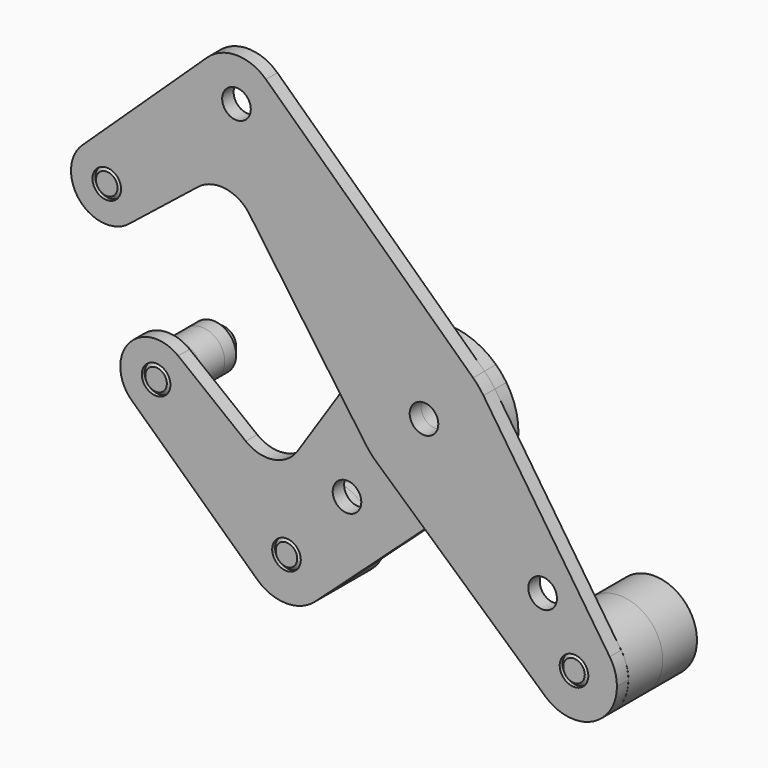
from build123d import *

# Parameters (mm, degrees)
F0_R      = 3.175
F0_R_2    = 3.96875
F2_DEPTH  = 3.175
F3_DEPTH  = 3.175
F4_R      = 9.525
F6_DEPTH  = 12.7
F4_R_2    = 5.08
F5_R      = 9.525
F5_R_2    = 5.08
F7_OFFSET = 0.0254
F8_SIZE   = 0.762
F8_2_SIZE = 0.762
F8_3_SIZE = 0.762
F8_4_SIZE = 0.762


with BuildPart() as f2:
    # F0 (on Front) → F2 (new body)
    with BuildSketch(Plane.XZ):
        with BuildLine():
            ThreePointArc((26.9262440233, -45.4676864135), (37.1682864336, -47.0737686401), (42.8102251661, -38.3762138003))
            ThreePointArc((42.8102251661, -38.3762138003), (42.3999454948, -35.6108027404), (41.2044512386, -33.0836262089))
            ThreePointArc((41.2044512386, -33.0836262089), (27.0442454474, -31.1806737127), (26.9262440233, -45.4676864135))
        make_face()
        with Locations((33.2852251661, -38.3762138003)):
            Circle(F0_R, mode=Mode.SUBTRACT)
        with BuildLine():
            ThreePointArc((-32.0815314576, 47.9702672503), (-32.8608164346, 51.7436071154), (-35.0711574392, 54.8995176744))
            ThreePointArc((-35.0711574392, 54.8995176744), (-41.6065314576, 57.4952672503), (-48.1419054761, 54.8995176744))
            ThreePointArc((-48.1419054761, 54.8995176744), (-45.3798713227, 39.2245522274), (-32.0815314576, 47.9702672503))
        make_face()
        with Locations((-41.6065314576, 47.9702672503)):
            Circle(F0_R, mode=Mode.SUBTRACT)
        with BuildLine():
            ThreePointArc((-62.4511918078, 23.0063483758), (-67.2442419203, 30.2944442282), (-75.8348368232, 28.7807237291))
            ThreePointArc((-75.8348368232, 28.7807237291), (-76.3849752141, 17.8055319436), (-65.4422370763, 16.798571653))
            ThreePointArc((-65.4422370763, 16.798571653), (-63.237943921, 19.5609585706), (-62.4511918078, 23.0063483758))
        make_face()
        with Locations((-70.3886918078, 23.0063483758)):
            Circle(F0_R, mode=Mode.SUBTRACT)
        with BuildLine():
            ThreePointArc((-12.9726166036, -9.1502373442), (-15.8730587934, -0.2482529814), (-13.2524193062, 8.7400805221))
            Line((-13.2524193062, 8.7400805221), (-19.2147683858, -0.3005169703))
            Line((-19.2147683858, -0.3005169703), (-12.9726166036, -9.1502373442))
        make_face()
        with BuildLine():
            Line((-10.5983019047, -11.8191210221), (0.0653932355, -21.3813431455))
            Line((0.0653932355, -21.3813431455), (10.6703987497, -11.7540722953))
            ThreePointArc((10.6703987497, -11.7540722953), (0.0485522706, -15.8749257534), (-10.5983019047, -11.8191210221))
        make_face()
        with BuildLine():
            ThreePointArc((26.9262440233, -45.4676864135), (27.0442454474, -31.1806737127), (41.2044512386, -33.0836262089))
            Line((41.2044512386, -33.0836262089), (13.1987101208, 8.820979319))
            ThreePointArc((13.1987101208, 8.820979319), (15.1912005478, 4.609018433), (15.875, 0))
            ThreePointArc((15.875, 0), (14.5156502636, -6.4274040191), (10.6703987497, -11.7540722953))
            Line((10.6703987497, -11.7540722953), (0.0653932355, -21.3813431455))
            Line((0.0653932355, -21.3813431455), (26.9262440233, -45.4676864135))
        make_face()
        with Locations((26.3222689506, -25.5025770961)):
            Circle(F0_R, mode=Mode.SUBTRACT)
        with BuildLine():
            ThreePointArc((-13.2524193062, 8.7400805221), (-1.834314477, 15.7686687897), (10.8922900307, 11.5487507067))
            Line((10.8922900307, 11.5487507067), (-35.0711574392, 54.8995176744))
            ThreePointArc((-35.0711574392, 54.8995176744), (-32.8608164346, 51.7436071154), (-32.0815314576, 47.9702672503))
            ThreePointArc((-32.0815314576, 47.9702672503), (-45.3798713227, 39.2245522274), (-48.1419054761, 54.8995176744))
            Line((-48.1419054761, 54.8995176744), (-75.8348368232, 28.7807237291))
            ThreePointArc((-75.8348368232, 28.7807237291), (-67.2442419203, 30.2944442282), (-62.4511918078, 23.0063483758))
            ThreePointArc((-62.4511918078, 23.0063483758), (-63.237943921, 19.5609585706), (-65.4422370763, 16.798571653))
            Line((-65.4422370763, 16.798571653), (-50.1509863937, 28.9828821829))
            ThreePointArc((-50.1509863937, 28.9828821829), (-44.0823996147, 30.6328866939), (-38.7182233604, 27.3502241323))
            Line((-38.7182233604, 27.3502241323), (-19.2147683858, -0.3005169703))
            Line((-19.2147683858, -0.3005169703), (-13.2524193062, 8.7400805221))
        make_face()
        with BuildLine():
            ThreePointArc((15.875, 0), (15.1912005478, 4.609018433), (13.1987101208, 8.820979319))
            ThreePointArc((13.1987101208, 8.820979319), (12.1224690662, 10.2499448164), (10.8922900307, 11.5487507067))
            ThreePointArc((10.8922900307, 11.5487507067), (-1.834314477, 15.7686687897), (-13.2524193062, 8.7400805221))
            ThreePointArc((-13.2524193062, 8.7400805221), (-15.8730587934, -0.2482529814), (-12.9726166036, -9.1502373442))
            ThreePointArc((-12.9726166036, -9.1502373442), (-11.8607666217, -10.5516747555), (-10.5983019047, -11.8191210221))
            ThreePointArc((-10.5983019047, -11.8191210221), (0.0485522706, -15.8749257534), (10.6703987497, -11.7540722953))
            ThreePointArc((10.6703987497, -11.7540722953), (14.5156502636, -6.4274040191), (15.875, 0))
        make_face()
        Circle(F0_R_2, mode=Mode.SUBTRACT)
        Circle(F0_R_2)
        Circle(F0_R, mode=Mode.SUBTRACT)
    extrude(amount=F2_DEPTH)


with BuildPart() as f3:
    # F0 (on Front) → F3 (new body)
    with BuildSketch(Plane.XZ):
        with BuildLine():
            ThreePointArc((15.875, 0), (15.1912005478, 4.609018433), (13.1987101208, 8.820979319))
            ThreePointArc((13.1987101208, 8.820979319), (12.1224690662, 10.2499448164), (10.8922900307, 11.5487507067))
            ThreePointArc((10.8922900307, 11.5487507067), (-1.834314477, 15.7686687897), (-13.2524193062, 8.7400805221))
            ThreePointArc((-13.2524193062, 8.7400805221), (-15.8730587934, -0.2482529814), (-12.9726166036, -9.1502373442))
            ThreePointArc((-12.9726166036, -9.1502373442), (-11.8607666217, -10.5516747555), (-10.5983019047, -11.8191210221))
            ThreePointArc((-10.5983019047, -11.8191210221), (0.0485522706, -15.8749257534), (10.6703987497, -11.7540722953))
            ThreePointArc((10.6703987497, -11.7540722953), (14.5156502636, -6.4274040191), (15.875, 0))
        make_face()
        Circle(F0_R_2, mode=Mode.SUBTRACT)
        with BuildLine():
            ThreePointArc((-12.9726166036, -9.1502373442), (-15.8730587934, -0.2482529814), (-13.2524193062, 8.7400805221))
            Line((-13.2524193062, 8.7400805221), (-19.2147683858, -0.3005169703))
            Line((-19.2147683858, -0.3005169703), (-12.9726166036, -9.1502373442))
        make_face()
        with BuildLine():
            Line((-10.5983019047, -11.8191210221), (0.0653932355, -21.3813431455))
            Line((0.0653932355, -21.3813431455), (10.6703987497, -11.7540722953))
            ThreePointArc((10.6703987497, -11.7540722953), (0.0485522706, -15.8749257534), (-10.5983019047, -11.8191210221))
        make_face()
        with BuildLine():
            ThreePointArc((-39.5427300894, -45.5481910186), (-33.1114263313, -48.1038957423), (-26.647623873, -45.6315380732))
            ThreePointArc((-26.647623873, -45.6315380732), (-24.3404729646, -42.4355371074), (-23.5248631228, -38.579094696))
            ThreePointArc((-23.5248631228, -38.579094696), (-36.849933329, -29.8449609995), (-39.5427300894, -45.5481910186))
        make_face()
        with Locations((-33.0498631228, -38.579094696)):
            Circle(F0_R, mode=Mode.SUBTRACT)
        with BuildLine():
            ThreePointArc((-57.0757936348, -7.5537803256), (-68.0121676911, -8.627656241), (-67.394906617, -19.5992776228))
            ThreePointArc((-67.394906617, -19.5992776228), (-58.817458973, -21.070142101), (-54.0466841448, -13.7916973539))
            ThreePointArc((-54.0466841448, -13.7916973539), (-54.8440071189, -10.3244537385), (-57.0757936348, -7.5537803256))
        make_face()
        with Locations((-61.9841841448, -13.7916973539)):
            Circle(F0_R, mode=Mode.SUBTRACT)
        with BuildLine():
            Line((-26.647623873, -45.6315380732), (0.0653932355, -21.3813431455))
            Line((0.0653932355, -21.3813431455), (-10.5983019047, -11.8191210221))
            ThreePointArc((-10.5983019047, -11.8191210221), (-11.8607666217, -10.5516747555), (-12.9726166036, -9.1502373442))
            Line((-12.9726166036, -9.1502373442), (-19.2147683858, -0.3005169703))
            Line((-19.2147683858, -0.3005169703), (-30.5474012326, -17.4839744853))
            ThreePointArc((-30.5474012326, -17.4839744853), (-35.9047663103, -20.9493627188), (-42.0820013957, -19.3518512525))
            Line((-42.0820013957, -19.3518512525), (-57.0757936348, -7.5537803256))
            ThreePointArc((-57.0757936348, -7.5537803256), (-54.8440071189, -10.3244537385), (-54.0466841448, -13.7916973539))
            ThreePointArc((-54.0466841448, -13.7916973539), (-58.817458973, -21.070142101), (-67.394906617, -19.5992776228))
            Line((-67.394906617, -19.5992776228), (-39.5427300894, -45.5481910186))
            ThreePointArc((-39.5427300894, -45.5481910186), (-36.849933329, -29.8449609995), (-23.5248631228, -38.579094696))
            ThreePointArc((-23.5248631228, -38.579094696), (-24.3404729646, -42.4355371074), (-26.647623873, -45.6315380732))
        make_face()
        with Locations((-19.6233562292, -22.9063374758)):
            Circle(F0_R, mode=Mode.SUBTRACT)
        Circle(F0_R_2)
        Circle(F0_R, mode=Mode.SUBTRACT)
    extrude(amount=-F3_DEPTH)


with BuildPart() as f6:
    # F4 (on face) → F6 (new body, through all)
    with BuildSketch(Plane.XZ.offset(3.175)):
        with Locations((33.2852251661, -38.3762138003)):
            Circle(F4_R)
    extrude(amount=-F6_DEPTH)

    # F7: cut F2, F3, each made larger all round first
    f7_tool = offset(f2.part, amount=F7_OFFSET, kind=Kind.INTERSECTION, mode=Mode.PRIVATE)
    add(f7_tool, mode=Mode.SUBTRACT)
    f7_tool1 = offset(f3.part, amount=F7_OFFSET, kind=Kind.INTERSECTION, mode=Mode.PRIVATE)
    add(f7_tool1, mode=Mode.SUBTRACT)

    # F8#4
    f8_4_edges = [f6.edges().sort_by_distance(p)[0] for p in [
        (30.135625, -3.175, -38.376214),
    ]]
    chamfer(f8_4_edges, length=F8_4_SIZE)



with BuildPart() as f6b:
    # F4 (on face) → F6, piece 2 (new body, through all)
    with BuildSketch(Plane.XZ.offset(3.175)):
        with Locations((-70.3886918078, 23.0063483758)):
            Circle(F4_R_2)
    extrude(amount=-F6_DEPTH)

    # F7: cut F2, F3, each made larger all round first
    f7_tool = offset(f2.part, amount=F7_OFFSET, kind=Kind.INTERSECTION, mode=Mode.PRIVATE)
    add(f7_tool, mode=Mode.SUBTRACT)
    f7_tool1 = offset(f3.part, amount=F7_OFFSET, kind=Kind.INTERSECTION, mode=Mode.PRIVATE)
    add(f7_tool1, mode=Mode.SUBTRACT)

    # F8
    f8_edges = [f6b.edges().sort_by_distance(p)[0] for p in [
        (-73.538292, -3.175, 23.006348),
    ]]
    chamfer(f8_edges, length=F8_SIZE)


with BuildPart() as f6c:
    # F5 (on face) → F6, piece 3 (new body, through all)
    with BuildSketch(Plane.XZ):
        with Locations((-33.0498631228, -38.579094696)):
            Circle(F5_R)
    extrude(amount=-F6_DEPTH)

    # F7: cut F2, F3, each made larger all round first
    f7_tool = offset(f2.part, amount=F7_OFFSET, kind=Kind.INTERSECTION, mode=Mode.PRIVATE)
    add(f7_tool, mode=Mode.SUBTRACT)
    f7_tool1 = offset(f3.part, amount=F7_OFFSET, kind=Kind.INTERSECTION, mode=Mode.PRIVATE)
    add(f7_tool1, mode=Mode.SUBTRACT)

    # F8#2
    f8_2_edges = [f6c.edges().sort_by_distance(p)[0] for p in [
        (-36.199463, 0, -38.579095),
    ]]
    chamfer(f8_2_edges, length=F8_2_SIZE)


with BuildPart() as f6d:
    # F5 (on face) → F6, piece 4 (new body, through all)
    with BuildSketch(Plane.XZ):
        with Locations((-61.9841841448, -13.7916973539)):
            Circle(F5_R_2)
    extrude(amount=-F6_DEPTH)

    # F7: cut F2, F3, each made larger all round first
    f7_tool = offset(f2.part, amount=F7_OFFSET, kind=Kind.INTERSECTION, mode=Mode.PRIVATE)
    add(f7_tool, mode=Mode.SUBTRACT)
    f7_tool1 = offset(f3.part, amount=F7_OFFSET, kind=Kind.INTERSECTION, mode=Mode.PRIVATE)
    add(f7_tool1, mode=Mode.SUBTRACT)

    # F8#3
    f8_3_edges = [f6d.edges().sort_by_distance(p)[0] for p in [
        (-65.133784, 0, -13.791697),
    ]]
    chamfer(f8_3_edges, length=F8_3_SIZE)


with BuildPart() as f6_1:
    add(f6.part)

    add(f6b.part)  # F9 merges F6b

    add(f6c.part)  # F9 merges F6c

    add(f6d.part)  # F9 merges F6d
    # F9: F6d, F6c, F6b, F6 across plane
    add(f6d.part.mirror(Plane.XZ.offset(-9.525)))
    add(f6c.part.mirror(Plane.XZ.offset(-9.525)))
    add(f6b.part.mirror(Plane.XZ.offset(-9.525)))
    add(f6.part.mirror(Plane.XZ.offset(-9.525)))


solid = Compound([f2.part, f3.part, f6_1.part])
